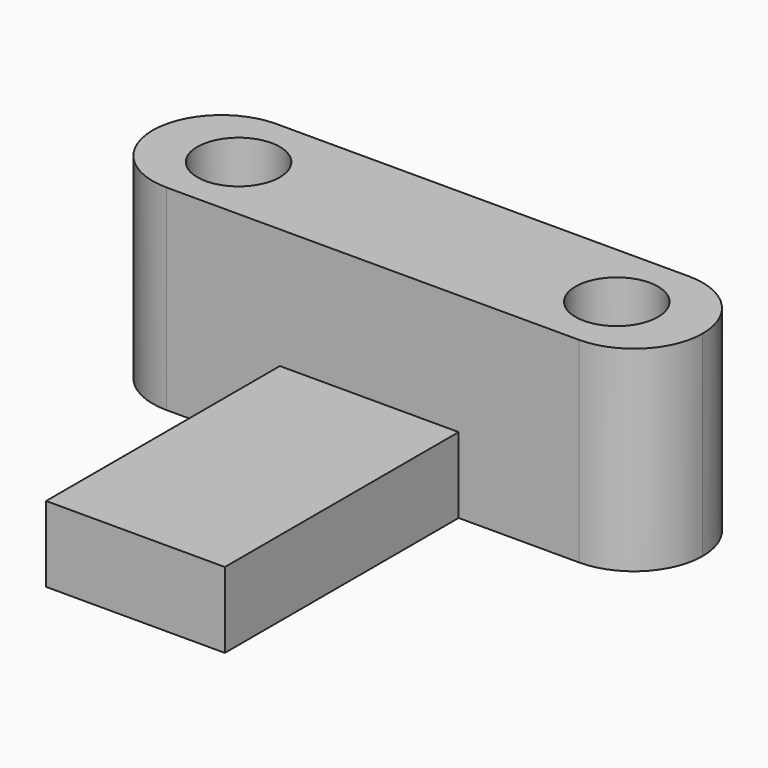
from build123d import *

# Parameters (mm, degrees)
F0_W          = 5.2
F0_H          = 2.2
F1_DEPTH      = 12.5
F2_W          = 5.2
F2_H          = 4
F3_DEPTH      = 3.5
F5_DEPTH      = 10.5
F5_DEPTH_BACK = 5.5
F7_DEPTH      = 5
F8_R          = 1.99999


# Not quite as in the source:
# - a fillet or chamfer is up to 0.001 mm smaller than in the source, because OpenCascade refuses the exact size


with BuildPart() as f1:
    # F0 (on Front) → F1 (new body)
    with BuildSketch(Plane.XZ):
        with Locations((-2.6, 1.1)):
            Rectangle(F0_W, F0_H)
    extrude(amount=-F1_DEPTH)

    # F2 (on face) → F3 (join)
    with BuildSketch(Plane.XY.offset(2.2)):
        with Locations((-2.6, 10.5)):
            Rectangle(F2_W, F2_H)
    extrude(amount=F3_DEPTH)

    # F4 (on face) → F5 (join, two sides)
    with BuildSketch(Plane.YZ) as f5_sk:
        Polygon((12.5, 0), (12.5, 5.7), (8.5, 5.7), (8.5, 2.2), (8.5, 0), align=None)
    extrude(amount=-F5_DEPTH)
    extrude(f5_sk.sketch, amount=F5_DEPTH_BACK)

    # F6 (on face) → F7 (cut)
    with BuildSketch(Plane.XY.offset(5.7)):
        with BuildLine():
            Line((-9.2, 10.5), (-8, 10.5))
            Line((-8, 10.5), (-6.8, 10.5))
            ThreePointArc((-6.8, 10.5), (-8, 11.7), (-9.2, 10.5))
        make_face()
        with BuildLine():
            Line((-6.8, 10.5), (-8, 10.5))
            Line((-8, 10.5), (-9.2, 10.5))
            ThreePointArc((-9.2, 10.5), (-8, 9.3), (-6.8, 10.5))
        make_face()
        with BuildLine():
            Line((3, 10.5), (1.8, 10.5))
            ThreePointArc((1.8, 10.5), (3, 9.3), (4.2, 10.5))
            Line((4.2, 10.5), (3, 10.5))
        make_face()
        with BuildLine():
            ThreePointArc((4.2, 10.5), (3, 11.7), (1.8, 10.5))
            Line((1.8, 10.5), (3, 10.5))
            Line((3, 10.5), (4.2, 10.5))
        make_face()
    extrude(amount=-F7_DEPTH, mode=Mode.SUBTRACT)

    # F8 (radius 2 in the source; OpenCascade refuses exactly that, so slightly less here)
    f8_edges = [f1.edges().sort_by_distance(p)[0] for p in [
        (5.5, 8.5, 2.85),
        (5.5, 12.5, 2.85),
        (-10.5, 12.5, 2.85),
        (-10.5, 8.5, 2.85),
    ]]
    fillet(f8_edges, radius=F8_R)


solid = f1.part
